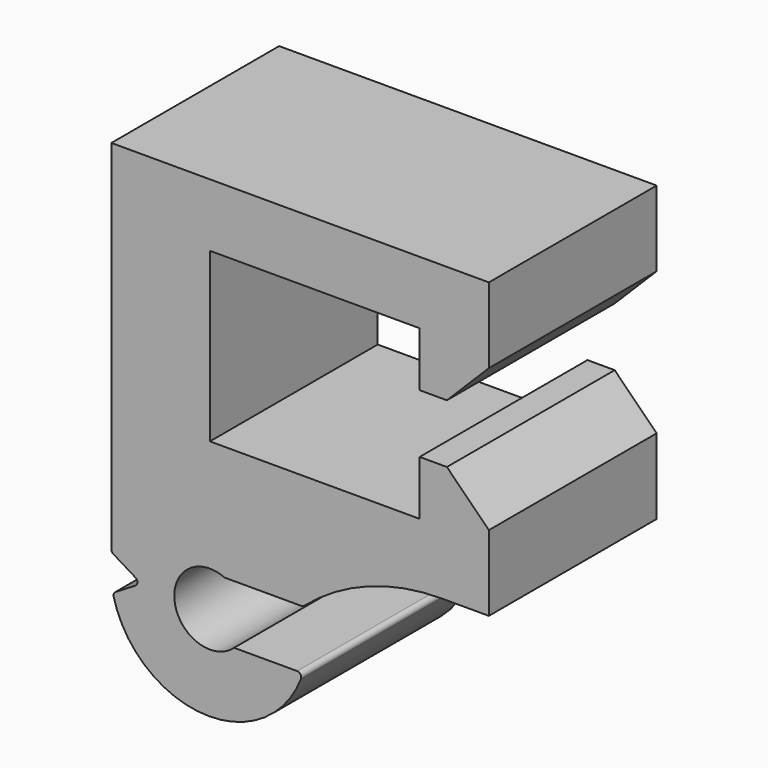
from build123d import *

# Parameters (mm, degrees)
F1_DEPTH    = 5
F2_SIZE     = 1
F3_T1_DEPTH = 5
F4_R        = 0.1


# Not quite as in the source:
# - a fillet or chamfer that OpenCascade refuses, or shapes differently, is made with other operations: its cross-section is extruded or revolved along the edge and cut away or added


with BuildPart() as f1:
    # F0 (on Front) → F1 (new body)
    with BuildSketch(Plane.XZ):
        with BuildLine():
            ThreePointArc((0.5760859311, -0.625), (-0.8390441156, -0.1360329819), (0.3491060011, 0.775))
            Line((0.3491060011, 0.775), (2.2185299187, 0.775))
            Line((2.2185299187, 0.775), (2.2185299187, 2.0197594836))
            Line((2.2185299187, 2.0197594836), (6.65, 2.0197594836))
            Line((6.65, 2.0197594836), (6.65, 4.8197594836))
            Line((6.65, 4.8197594836), (5, 4.8197594836))
            Line((5, 4.8197594836), (5, 3.5197594836))
            Line((5, 3.5197594836), (0, 3.5197594836))
            Line((0, 3.5197594836), (0, 7.5197594836))
            Line((0, 7.5197594836), (5, 7.5197594836))
            Line((5, 7.5197594836), (5, 6.2197594836))
            Line((5, 6.2197594836), (6.65, 6.2197594836))
            Line((6.65, 6.2197594836), (6.65, 9.0197594836))
            Line((6.65, 9.0197594836), (-2.35, 9.0197594836))
            Line((-2.35, 9.0197594836), (-2.35, 0.4335492267))
            Line((-2.35, 0.4335492267), (-1.6366346435, 0))
            Line((-1.6366346435, 0), (-2.3136941642, -0.4114842822))
            ThreePointArc((-2.3136941642, -0.4114842822), (-0.1293198619, -2.2532607786), (2.2185299187, -0.625))
            Line((2.2185299187, -0.625), (0.5760859311, -0.625))
        make_face()
    extrude(amount=F1_DEPTH)

    # F2
    f2_edges = [f1.edges().sort_by_distance(p)[0] for p in [
        (6.65, -2.5, 6.219759),
        (6.65, -2.5, 4.819759),
    ]]
    chamfer(f2_edges, length=F2_SIZE)

    # F3: fillet of radius 5 on 1 edges, made by hand

    # F3_s2 → F3_t1 (join)
    with BuildSketch(Plane.XZ):
        with BuildLine():
            ThreePointArc((5.5197673631, 2.0197594836), (3.7557099068, 1.6982315944), (2.2185299187, 0.775))
            Line((2.2185299187, 0.775), (2.2185299187, 2.0197594836))
            Line((2.2185299187, 2.0197594836), (5.5197673631, 2.0197594836))
        make_face()
    extrude(amount=F3_T1_DEPTH)

    # F4
    f4_edges = [f1.edges().sort_by_distance(p)[0] for p in [
        (-1.636635, -2.5, 0),
        (-2.313694, -2.5, -0.411484),
        (-2.35, -2.5, 0.433549),
        (2.21853, -2.5, -0.625),
        (2.21853, -2.5, 0.775),
    ]]
    fillet(f4_edges, radius=F4_R)


solid = f1.part
